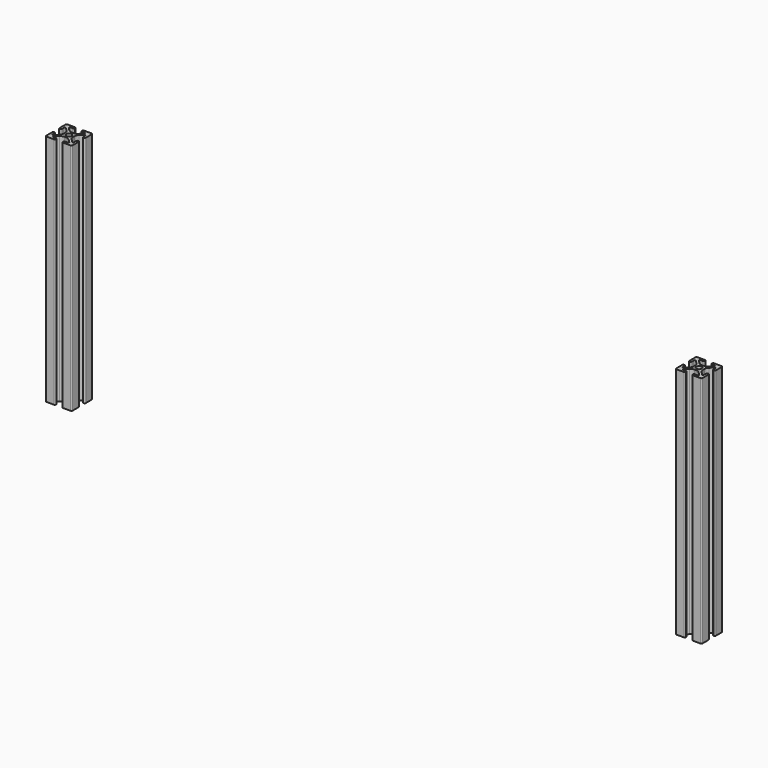
from build123d import *

# Parameters (mm, degrees)
F0_R     = 2.6035
F1_DEPTH = 226.06
F2_R     = 1.18109
F3_R     = 5.08
F4_R     = 0.762
F5_R     = 1.27


# Not quite as in the source:
# - a fillet or chamfer is up to 0.001 mm smaller than in the source, because OpenCascade refuses the exact size


with BuildPart() as f1:
    # F0 (on Top) → F1 (new body)
    with BuildSketch(Plane.XY):
        Polygon((12.7, 3.2385), (12.7, 12.7), (3.2385, 12.7), (3.2385, 10.3378), (8.7752354349, 10.3378), (2.9459354349, 4.5085), (-2.9459354349, 4.5085), (-8.7752354349, 10.3378), (-3.2385, 10.3378), (-3.2385, 12.7), (-12.7, 12.7), (-12.7, 3.2385), (-10.3378, 3.2385), (-10.3378, 8.7752354349), (-4.5085, 2.9459354349), (-4.5085, -2.9459354349), (-10.3378, -8.7752354349), (-10.3378, -3.2385), (-12.7, -3.2385), (-12.7, -12.7), (-3.2385, -12.7), (-3.2385, -10.3378), (-8.7752354349, -10.3378), (-2.9459354349, -4.5085), (2.9459354349, -4.5085), (8.7752354349, -10.3378), (3.2385, -10.3378), (3.2385, -12.7), (12.7, -12.7), (12.7, -3.2385), (10.3378, -3.2385), (10.3378, -8.7752354349), (4.5085, -2.9459354349), (4.5085, 2.9459354349), (10.3378, 8.7752354349), (10.3378, 3.2385), align=None)
        Circle(F0_R, mode=Mode.SUBTRACT)
    extrude(amount=F1_DEPTH)

    # F2 (radius 1.1811 in the source; OpenCascade refuses exactly that, so slightly less here)
    f2_edges = [f1.edges().sort_by_distance(p)[0] for p in [
        (3.2385, 12.7, 113.03),
        (3.2385, 10.3378, 113.03),
        (-3.2385, 12.7, 113.03),
        (-12.7, 3.2385, 113.03),
        (-3.2385, 10.3378, 113.03),
        (-10.3378, 3.2385, 113.03),
        (12.7, 3.2385, 113.03),
        (10.3378, 3.2385, 113.03),
        (12.7, -3.2385, 113.03),
        (10.3378, -3.2385, 113.03),
        (3.2385, -10.3378, 113.03),
        (-3.2385, -10.3378, 113.03),
        (-10.3378, -3.2385, 113.03),
        (-12.7, -3.2385, 113.03),
        (-3.2385, -12.7, 113.03),
        (3.2385, -12.7, 113.03),
    ]]
    fillet(f2_edges, radius=F2_R)

    # F3
    f3_edges = [f1.edges().sort_by_distance(p)[0] for p in [
        (2.945935, 4.5085, 113.03),
        (-2.945935, 4.5085, 113.03),
        (4.5085, -2.945935, 113.03),
        (4.5085, 2.945935, 113.03),
        (2.945935, -4.5085, 113.03),
        (-2.945935, -4.5085, 113.03),
        (-4.5085, -2.945935, 113.03),
        (-4.5085, 2.945935, 113.03),
    ]]
    fillet(f3_edges, radius=F3_R)

    # F4
    f4_edges = [f1.edges().sort_by_distance(p)[0] for p in [
        (8.775235, 10.3378, 113.03),
        (-8.775235, 10.3378, 113.03),
        (-10.3378, 8.775235, 113.03),
        (-10.3378, -8.775235, 113.03),
        (-8.775235, -10.3378, 113.03),
        (8.775235, -10.3378, 113.03),
        (10.3378, -8.775235, 113.03),
        (10.3378, 8.775235, 113.03),
    ]]
    fillet(f4_edges, radius=F4_R)

    # F5
    f5_edges = [f1.edges().sort_by_distance(p)[0] for p in [
        (-12.7, -12.7, 113.03),
        (12.7, -12.7, 113.03),
        (12.7, 12.7, 113.03),
        (-12.7, 12.7, 113.03),
    ]]
    fillet(f5_edges, radius=F5_R)


with BuildPart() as f6_1:
    # F6: copy of F1
    add(f1.part.moved(Location((609.6, 0, 0))))


solid = Compound([f1.part, f6_1.part])
